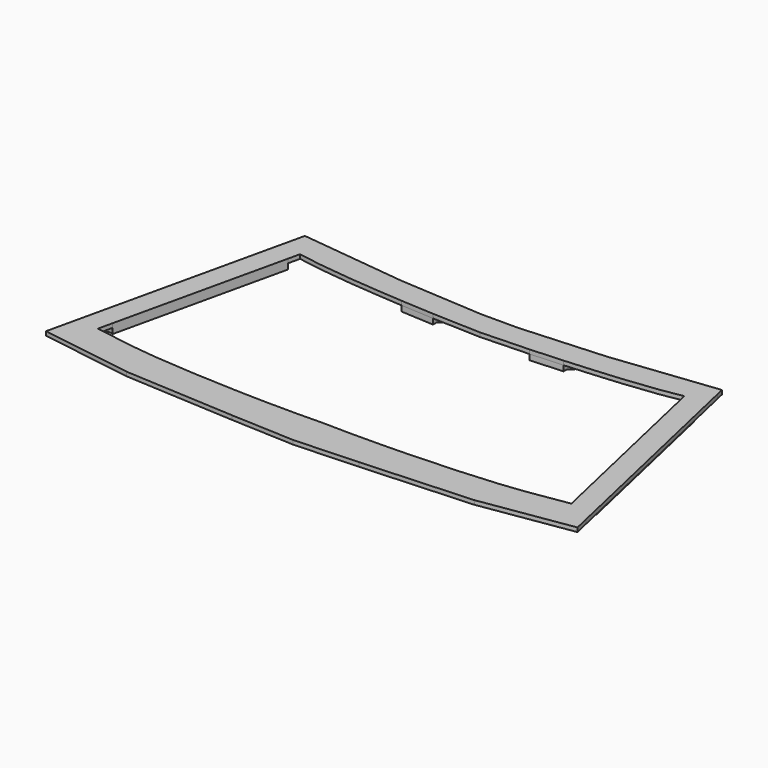
from build123d import *

# Parameters (mm, degrees)
F1_DEPTH = 0.75
F2_DEPTH = 1
F4_DEPTH = 0.75
F6_DEPTH = 0.75
F8_DEPTH = 0.75


with BuildPart() as f1:
    # F0 (on Top) → F1 (new body)
    with BuildSketch(Plane.XY):
        with BuildLine():
            add(Edge.make_bspline(
                [(-37.5, 18.7313321615), (-32.3807911431, 17.926577975), (-18.7011737223, 16.5680764405), (-7.3513992733, 15.9357535011), (0, 15.7313321615)],
                knots=[0, 0, 0, 0, 0.4901565124, 1, 1, 1, 1], degree=3))
            Line((-37.5, 18.7313321615), (-47, -23.1548529118))
            Line((-47, -23.1548529118), (-16.0084403101, -23.1548529118))
            Line((-16.0084403101, -23.1548529118), (-16.0063231241, -23.0646254072))
            add(Edge.make_bspline(
                [(-43.315390494, -20.4723017862), (-38.3905339247, -21.2993483436), (-33.0056838871, -22.2189238519), (-21.2861009313, -22.8925835376), (-16.0063231241, -23.0646254072)],
                knots=[0, 0, 0, 0, 0.398937465, 0.6969379575, 0.6969379575, 0.6969379575, 0.6969379575], degree=3))
            Line((-43.315390494, -20.4723017862), (-42.7131794367, -17.8171098074))
            Line((-42.7131794367, -17.8171098074), (-43.4446029246, -17.651219237))
            Line((-43.4446029246, -17.651219237), (-36.3666052528, 13.5561829132))
            Line((-36.3666052528, 13.5561829132), (-35.635181765, 13.3902923427))
            Line((-35.635181765, 13.3902923427), (-35.1425150574, 15.562495384))
            add(Edge.make_bspline(
                [(-35.1425150574, 15.562495384), (-30.4836686701, 14.6303577349), (-22.7091897663, 13.9291012054), (-15.9390947662, 13.4553124867), (-14.8013141006, 13.3810050341)],
                knots=[0, 0, 0, 0, 0.4908367268, 0.5909725979, 0.5909725979, 0.5909725979, 0.5909725979], degree=3))
            Line((-14.8013141006, 13.3810050341), (-14.8013141006, 14.1310050341))
            Line((-14.8013141006, 14.1310050341), (-8.8108518429, 13.792830613))
            Line((-8.8108518429, 13.792830613), (-8.8108518429, 13.042830613))
            add(Edge.make_bspline(
                [(-8.8108518429, 13.042830613), (-6.0913133604, 12.9141276056), (-3.2370188614, 12.8126642043), (0, 12.7313321615)],
                knots=[0.7661743328, 0.7661743328, 0.7661743328, 0.7661743328, 1, 1, 1, 1], degree=3))
            Line((0, 12.7313321615), (0, 15.7313321615))
        make_face()
        with BuildLine():
            Line((-16.0084403101, -23.1548529118), (-47, -23.1548529118))
            add(Edge.make_bspline(
                [(-47, -23.1548529118), (-39.471310208, -24.0545421828), (-29.2503257197, -25.7571688291), (-8.0323131497, -26.1634826516), (0, -26.1548529118)],
                knots=[0, 0, 0, 0, 0.4528935937, 1, 1, 1, 1], degree=3))
            Line((0, -26.1548529118), (0, -23.1548529118))
            add(Edge.make_bspline(
                [(-10.0079742572, -23.2053765011), (-6.5667353079, -23.2536816802), (-3.1521121944, -23.2431206783), (0, -23.1548529118)],
                knots=[0.8085428965, 0.8085428965, 0.8085428965, 0.8085428965, 1, 1, 1, 1], degree=3))
            Line((-10.0079742572, -23.2053765011), (-10.0255681439, -23.9551701095))
            Line((-10.0255681439, -23.9551701095), (-16.0239170108, -23.8144190156))
            Line((-16.0239170108, -23.8144190156), (-16.0084403101, -23.1548529118))
        make_face()
        with BuildLine():
            Line((-16.0063231241, -23.0646254072), (-16.0084403101, -23.1548529118))
            Line((-16.0084403101, -23.1548529118), (-12.748052928, -23.1548529118))
            add(Edge.make_bspline(
                [(-16.0063231241, -23.0646254072), (-14.9289009553, -23.0997332718), (-13.8402912127, -23.1300103495), (-12.748052928, -23.1548529118)],
                knots=[0.6969379575, 0.6969379575, 0.6969379575, 0.6969379575, 0.7577496714, 0.7577496714, 0.7577496714, 0.7577496714], degree=3))
        make_face()
        with BuildLine():
            Line((-12.748052928, -23.1548529118), (-16.0084403101, -23.1548529118))
            Line((-16.0084403101, -23.1548529118), (-16.0239170108, -23.8144190156))
            Line((-16.0239170108, -23.8144190156), (-10.0255681439, -23.9551701095))
            Line((-10.0255681439, -23.9551701095), (-10.0079742572, -23.2053765011))
            add(Edge.make_bspline(
                [(-12.748052928, -23.1548529118), (-11.8357565687, -23.1756027605), (-10.9209287599, -23.192561224), (-10.0079742572, -23.2053765011)],
                knots=[0.7577496714, 0.7577496714, 0.7577496714, 0.7577496714, 0.8085428965, 0.8085428965, 0.8085428965, 0.8085428965], degree=3))
        make_face()
        with BuildLine():
            add(Edge.make_bspline(
                [(-14.8013141006, 13.3810050341), (-12.8106074305, 13.2509937357), (-10.8485573953, 13.1392656642), (-8.8108518429, 13.042830613)],
                knots=[0.5909725979, 0.5909725979, 0.5909725979, 0.5909725979, 0.7661743328, 0.7661743328, 0.7661743328, 0.7661743328], degree=3))
            Line((-8.8108518429, 13.042830613), (-8.8108518429, 13.792830613))
            Line((-8.8108518429, 13.792830613), (-14.8013141006, 14.1310050341))
            Line((-14.8013141006, 14.1310050341), (-14.8013141006, 13.3810050341))
        make_face()
        Polygon((-43.4446029246, -17.651219237), (-42.7131794367, -17.8171098074), (-35.635181765, 13.3902923427), (-36.3666052528, 13.5561829132), align=None)
    extrude(amount=F1_DEPTH)

    # F0 (on Top) → F2 (join)
    with BuildSketch(Plane.XY):
        with BuildLine():
            Line((-16.0063231241, -23.0646254072), (-16.0084403101, -23.1548529118))
            Line((-16.0084403101, -23.1548529118), (-12.748052928, -23.1548529118))
            add(Edge.make_bspline(
                [(-16.0063231241, -23.0646254072), (-14.9289009553, -23.0997332718), (-13.8402912127, -23.1300103495), (-12.748052928, -23.1548529118)],
                knots=[0.6969379575, 0.6969379575, 0.6969379575, 0.6969379575, 0.7577496714, 0.7577496714, 0.7577496714, 0.7577496714], degree=3))
        make_face()
        with BuildLine():
            Line((-12.748052928, -23.1548529118), (-16.0084403101, -23.1548529118))
            Line((-16.0084403101, -23.1548529118), (-16.0239170108, -23.8144190156))
            Line((-16.0239170108, -23.8144190156), (-10.0255681439, -23.9551701095))
            Line((-10.0255681439, -23.9551701095), (-10.0079742572, -23.2053765011))
            add(Edge.make_bspline(
                [(-12.748052928, -23.1548529118), (-11.8357565687, -23.1756027605), (-10.9209287599, -23.192561224), (-10.0079742572, -23.2053765011)],
                knots=[0.7577496714, 0.7577496714, 0.7577496714, 0.7577496714, 0.8085428965, 0.8085428965, 0.8085428965, 0.8085428965], degree=3))
        make_face()
        with BuildLine():
            add(Edge.make_bspline(
                [(-14.8013141006, 13.3810050341), (-12.8106074305, 13.2509937357), (-10.8485573953, 13.1392656642), (-8.8108518429, 13.042830613)],
                knots=[0.5909725979, 0.5909725979, 0.5909725979, 0.5909725979, 0.7661743328, 0.7661743328, 0.7661743328, 0.7661743328], degree=3))
            Line((-8.8108518429, 13.042830613), (-8.8108518429, 13.792830613))
            Line((-8.8108518429, 13.792830613), (-14.8013141006, 14.1310050341))
            Line((-14.8013141006, 14.1310050341), (-14.8013141006, 13.3810050341))
        make_face()
        Polygon((-43.4446029246, -17.651219237), (-42.7131794367, -17.8171098074), (-35.635181765, 13.3902923427), (-36.3666052528, 13.5561829132), align=None)
    extrude(amount=-F2_DEPTH)

    # F3 (on face) → F4 (join, through all)
    with BuildSketch(Plane.XY.offset(0.75)):
        Polygon((-47.9752313172, -22.9336654846), (-47, -23.1548529118), (-37.5, 18.7313321615), (-38.4752313172, 18.9525195888), align=None)
    extrude(amount=-F4_DEPTH)

    # F5 (on face) → F6 (join, through all)
    with BuildSketch(Plane.XY.offset(0.75)):
        with BuildLine():
            Line((-38.1434501763, 20.4153665646), (-38.4752313172, 18.9525195888))
            Line((-38.4752313172, 18.9525195888), (-37.5, 18.7313321615))
            add(Edge.make_bspline(
                [(-37.5, 18.7313321615), (-32.3807911431, 17.926577975), (-18.7011737223, 16.5680764405), (-7.3513992733, 15.9357535011), (0, 15.7313321615)],
                knots=[0, 0, 0, 0, 0.4901565124, 1, 1, 1, 1], degree=3))
            Line((0, 15.7313321615), (0, 17.2313321615))
            Line((0, 17.2313321615), (-3.3217752352, 17.2313321615))
            Line((-3.3217752352, 17.2313321615), (-18.8273077893, 18.2105369309))
            Line((-18.8273077893, 18.2105369309), (-38.1434501763, 20.4153665646))
        make_face()
    extrude(amount=-F6_DEPTH)

    # F7 (on face) → F8 (join, through all)
    with BuildSketch(Plane.XY.offset(0.75)):
        with BuildLine():
            Line((-47, -23.1548529118), (-47.9752313172, -22.9336654846))
            Line((-47.9752313172, -22.9336654846), (-48.6002014355, -25.6892038047))
            Line((-48.6002014355, -25.6892038047), (-31.8084545434, -28.2887462527))
            Line((-31.8084545434, -28.2887462527), (-11.6026224568, -29.4112917036))
            Line((-11.6026224568, -29.4112917036), (0, -29.9293901771))
            Line((0, -29.9293901771), (0, -26.1548529118))
            add(Edge.make_bspline(
                [(-47, -23.1548529118), (-39.471310208, -24.0545421828), (-29.2503257197, -25.7571688291), (-8.0323131497, -26.1634826516), (0, -26.1548529118)],
                knots=[0, 0, 0, 0, 0.4528935937, 1, 1, 1, 1], degree=3))
        make_face()
    extrude(amount=-F8_DEPTH)

    # F9 (on face) → F11 section 0
    with BuildSketch(Plane.YZ.offset(-8.8108518429)):
        Polygon((13.792830613, -0.5), (13.792830613, -1), (15.6468802348, -1.75), (15.6468802348, -1.25), align=None)
    # F10 (on face) → F11 section 1
    with BuildSketch(Plane(origin=(-14.8013141006, 0, 0), x_dir=(0, -1, 0), z_dir=(-1, 0, 0))):
        Polygon((-15.9850546559, -1.75), (-14.1310050341, -1), (-14.1310050341, -0.5), (-15.9850546559, -1.25), align=None)
    loft()

    # F12 (on face) → F14 section 0
    with BuildSketch(Plane(origin=(-15.4566018313, 0.3626887438, 0), x_dir=(-0.0234585156, -0.9997248112, 0), z_dir=(-0.9997248112, 0.0234585156, 0))):
        Polygon((24.1837628611, -0.5), (24.1837628611, -1), (26.0378124829, -1.75), (26.0378124829, -1.25), align=None)
    # F13 (on face) → F14 section 1
    with BuildSketch(Plane(origin=(-9.4582529644, 0.2219376499, 0), x_dir=(0.0234585156, 0.9997248112, 0), z_dir=(0.9997248112, -0.0234585156, 0))):
        Polygon((-26.0378124829, -1.75), (-24.1837628611, -1), (-24.1837628611, -0.5), (-26.0378124829, -1.25), align=None)
    loft()

    # F15 (on face) → F17 section 0
    with BuildSketch(Plane(origin=(1.1449940284, 5.04836124, 0), x_dir=(-0.9752313172, 0.2211874272, 0), z_dir=(0.2211874272, 0.9752313172, 0))):
        Polygon((38.4643095643, -0.5), (38.4643095643, -1), (40.3183591861, -1.75), (40.3183591861, -1.25), align=None)
    # F16 (on face) → F17 section 1
    with BuildSketch(Plane(origin=(-5.9330036433, -26.1590409101, 0), x_dir=(0.9752313172, -0.2211874272, 0), z_dir=(-0.2211874272, -0.9752313172, 0))):
        Polygon((-40.3183591861, -1.75), (-38.4643095643, -1), (-38.4643095643, -0.5), (-40.3183591861, -1.25), align=None)
    loft()

    # F18: F1 across plane


with BuildPart() as f1_1:
    add(f1.part)
    add(f1.part.mirror(Plane.YZ))


solid = f1_1.part
